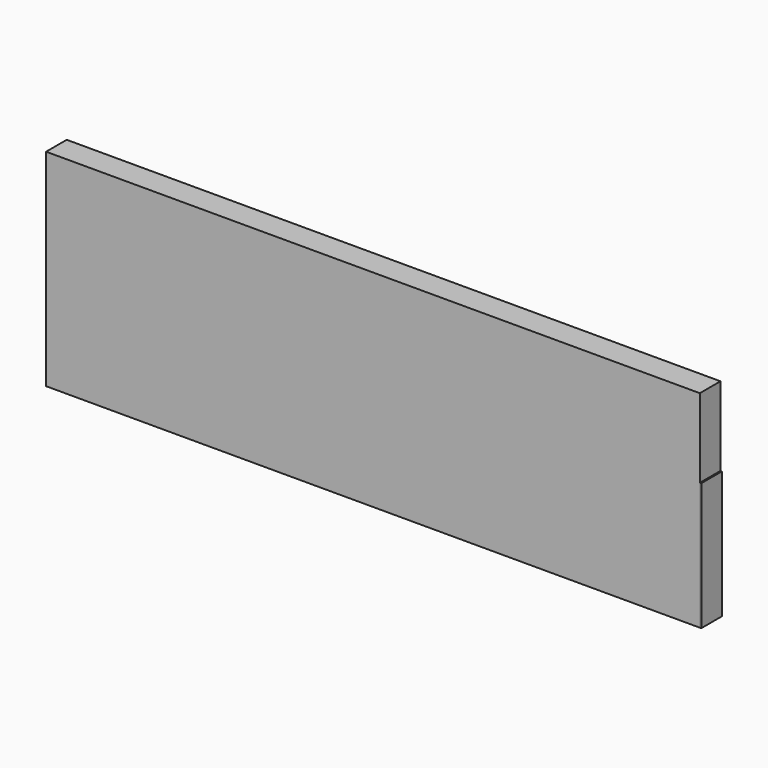
from build123d import *

# Parameters (mm, degrees)
F2_DEPTH = 2.38125
F0_W     = 60.325
F0_H     = 19.05


# Not quite as in the source:
# - a feature of the source that left no trace in its solid (it failed there, or was rolled back) is left out


with BuildPart() as f2:
    # F1 (on Front) → F2 (new body)
    with BuildSketch(Plane.XZ):
        with BuildLine():
            ThreePointArc((12.0106148621, 7.2541593159), (15.4199186631, 2.407427548), (19.84375, 6.35))
            ThreePointArc((19.84375, 6.35), (18.8687445476, 8.9554692756), (16.4227886665, 10.2807638112))
            ThreePointArc((16.4227886665, 10.2807638112), (13.7755602888, 9.4105561157), (12.0106148621, 7.2541593159))
        make_face()
        with BuildLine():
            ThreePointArc((16.4227886665, 10.2807638112), (18.8687445476, 8.9554692756), (19.84375, 6.35))
            ThreePointArc((19.84375, 6.35), (15.4199186631, 2.407427548), (12.0106148621, 7.2541593159))
            Line((12.0106148621, 7.2541593159), (8.8399816304, 0))
            Line((8.8399816304, 0), (60.4599677026, 0))
            Line((60.4599677026, 0), (60.4599677026, 11.7762926966))
            Line((60.4599677026, 11.7762926966), (16.4227886665, 10.2807638112))
        make_face()
        with BuildLine():
            ThreePointArc((12.0106148621, 7.2541593159), (13.7755602888, 9.4105561157), (16.4227886665, 10.2807638112))
            ThreePointArc((16.4227886665, 10.2807638112), (13.6299973872, 9.6227572216), (12.0106148621, 7.2541593159))
        make_face()
    extrude(amount=F2_DEPTH)


with BuildPart() as f2b:
    # F0 (on Front) → F2, piece 2 (new body)
    with BuildSketch(Plane.XZ):
        with Locations((30.1625, 9.525)):
            Rectangle(F0_W, F0_H)
    extrude(amount=F2_DEPTH)


solid = Compound([f2.part, f2b.part])
